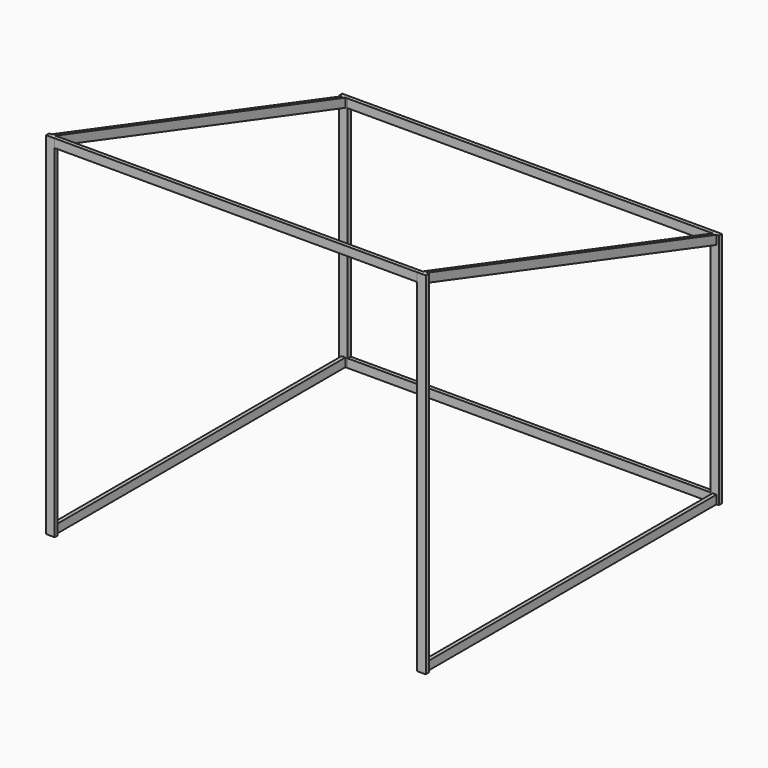
from build123d import *

# Parameters (mm, degrees)
F1_W          = 90
F1_H          = 3700
F2_DEPTH      = 40
F3_W          = 3820
F3_H          = 90
F4_DEPTH      = 40
F8_DEPTH      = 20
F8_DEPTH_BACK = 20
F7_W          = 3820
F7_H          = 90
F10_W         = 90
F10_H         = 2500
F11_DEPTH     = 40
F10_W_2       = 3819.998
F10_H_2       = 90


with BuildPart() as f2:
    # F1 (on Front) → F2 (new body)
    with BuildSketch(Plane.XZ):
        with Locations((-1955, 0)):
            Rectangle(F1_W, F1_H)
    extrude(amount=F2_DEPTH)


with BuildPart() as f2b:
    # F1 (on Front) → F2, piece 2 (new body)
    with BuildSketch(Plane.XZ):
        with Locations((1955, 0)):
            Rectangle(F1_W, F1_H)
    extrude(amount=F2_DEPTH)

    # F9: F8, F8b across plane


with BuildPart() as f4:
    # F3 (on face) → F4 (new body)
    with BuildSketch(Plane.XZ):
        with Locations((0, 1805)):
            Rectangle(F3_W, F3_H)
    extrude(amount=F4_DEPTH)


with BuildPart() as f8:
    # F7 (on offset) → F8 (new body, two sides)
    with BuildSketch(Plane(origin=(-1955, 0, 0), x_dir=(0, -1, 0), z_dir=(-1, 0, 0))) as f8_sk:
        Polygon((0, 1755.6637917124), (0, 1850), (-3820, 650), (-3820, 555.6637917124), align=None)
    extrude(amount=F8_DEPTH)
    extrude(f8_sk.sketch, amount=-F8_DEPTH_BACK)


with BuildPart() as f8b:
    # F7 (on offset) → F8, piece 2 (new body, two sides)
    with BuildSketch(Plane(origin=(-1955, 0, 0), x_dir=(0, -1, 0), z_dir=(-1, 0, 0))) as f8_2_sk:
        with Locations((-1910, -1805)):
            Rectangle(F7_W, F7_H)
    extrude(amount=F8_DEPTH)
    extrude(f8_2_sk.sketch, amount=-F8_DEPTH_BACK)


with BuildPart() as f2b_1:
    add(f2b.part)
    add(f8.part.mirror(Plane.YZ))
    add(f8b.part.mirror(Plane.YZ))


with BuildPart() as f11:
    # F10 (on face) → F11 (new body)
    with BuildSketch(Plane(origin=(0, 3820, 0), x_dir=(-1, 0, 0), z_dir=(0, 1, 0))):
        with Locations((-1955, -600)):
            Rectangle(F10_W, F10_H)
    extrude(amount=F11_DEPTH)


with BuildPart() as f11b:
    # F10 (on face) → F11, piece 2 (new body)
    with BuildSketch(Plane(origin=(0, 3820, 0), x_dir=(-1, 0, 0), z_dir=(0, 1, 0))):
        with Locations((1955, -600)):
            Rectangle(F10_W, F10_H)
    extrude(amount=F11_DEPTH)


with BuildPart() as f11c:
    # F10 (on face) → F11, piece 3 (new body)
    with BuildSketch(Plane(origin=(0, 3820, 0), x_dir=(-1, 0, 0), z_dir=(0, 1, 0))):
        with Locations((0, 605)):
            Rectangle(F10_W_2, F10_H_2)
    extrude(amount=F11_DEPTH)


with BuildPart() as f11d:
    # F10 (on face) → F11, piece 4 (new body)
    with BuildSketch(Plane(origin=(0, 3820, 0), x_dir=(-1, 0, 0), z_dir=(0, 1, 0))):
        with Locations((0, -1805)):
            Rectangle(F10_W_2, F10_H_2)
    extrude(amount=F11_DEPTH)


solid = Compound([f2.part, f4.part, f8.part, f8b.part, f2b_1.part, f11.part, f11b.part, f11c.part, f11d.part])
